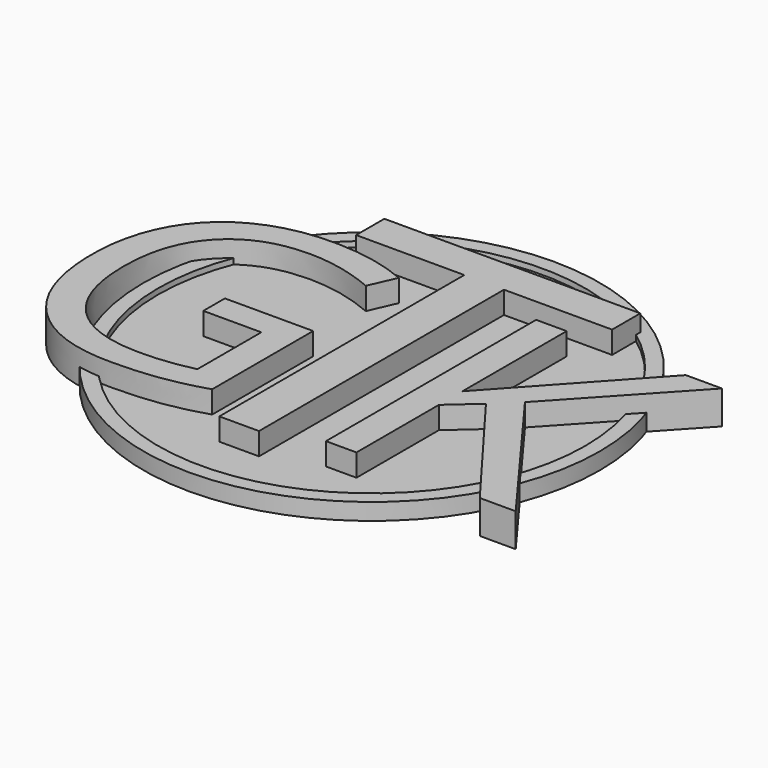
from build123d import *

# Parameters (mm, degrees)
F0_TEXT_SIZE   = 65.2506119675
F0_TEXT_SIZE_2 = 66.0528739293
F0_TEXT_SIZE_3 = 85.8419936978
F1_DEPTH       = 6
F2_R           = 40.9488233013
F2_R_2         = 38.3242145181
F3_DEPTH       = 3
F4_DEPTH       = 2
F7_R           = 2.5
F8_DEPTH       = 12.5


# Not quite as in the source:
# - Text() gives the source's letters only with a copy of the font that has no kerning and outlines rounded to 1/6400 em; it was checked with that copy


with BuildPart() as f1:
    # F0 (on Top) → F1 (new body)
    with BuildSketch(Plane.XY):
        with Locations((-52.7567267418, -32.1546457708)):
            Text('G', F0_TEXT_SIZE, font='Open Sans', text_align=(TextAlign.LEFT, TextAlign.BOTTOM))
        with Locations((5.7762847282, -32.7322743833)):
            Text('K', F0_TEXT_SIZE_2, font='Open Sans', text_align=(TextAlign.LEFT, TextAlign.BOTTOM))
        with Locations((-24.2603914812, -36.1980460584)):
            Text('T', F0_TEXT_SIZE_3, font='Open Sans', text_align=(TextAlign.LEFT, TextAlign.BOTTOM))
    extrude(amount=F1_DEPTH)


with BuildPart() as f3:
    # F2 (on Top) → F3 (new body)
    with BuildSketch(Plane.XY):
        with Locations((-74.4824782014, 97.6905226707)):
            Circle(F2_R)
        with Locations((-74.4824782014, 97.6905226707)):
            Circle(F2_R_2, mode=Mode.SUBTRACT)
    extrude(amount=F3_DEPTH)


with BuildPart() as f4:
    # F2 (on Top) → F4 (new body)
    with BuildSketch(Plane.XY):
        with Locations((-74.4824782014, 97.6905226707)):
            Circle(F2_R_2)
    extrude(amount=F4_DEPTH)


with BuildPart() as f3_1:
    # F5: moved
    add(f3.part.moved(Location((74.10387, -104.36464, 0))))


with BuildPart() as f4_1:
    # F6: moved
    add(f4.part.moved(Location((74.10387, -104.36464, 0))))


with BuildPart() as f8:
    # F7 (on Top) → F8 (new body, symmetric)
    with BuildSketch(Plane.XY):
        with Locations((0, 28.1020509964)):
            Circle(F7_R)
    extrude(amount=F8_DEPTH, both=True)


with BuildPart() as f4_2:
    add(f4_1.part)

    # F9: cut F8
    add(f8.part, mode=Mode.SUBTRACT)


solid = Compound([f1.part, f3_1.part, f4_2.part])
